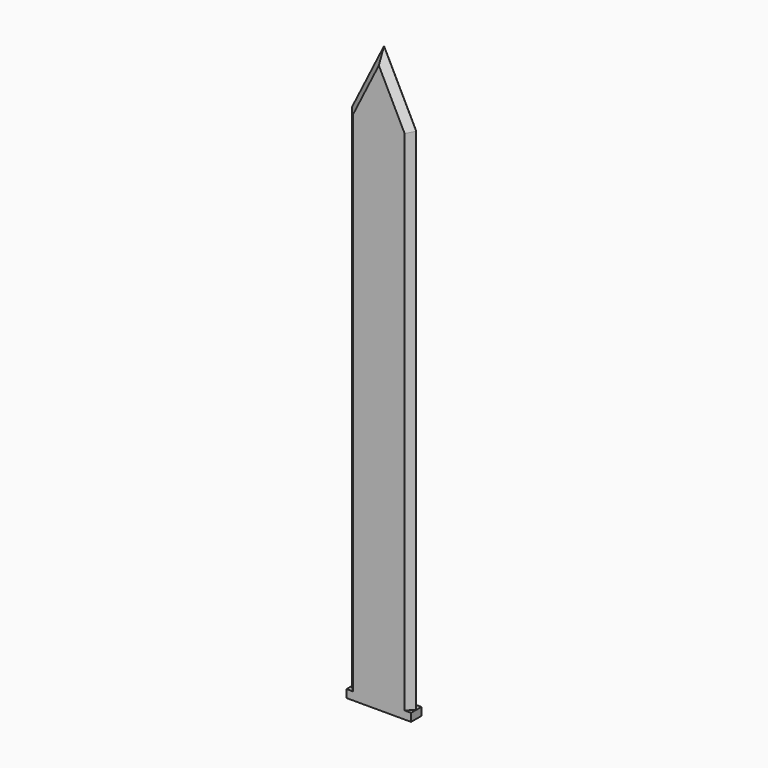
from build123d import *

# Parameters (mm, degrees)
F0_W     = 76.2
F0_H     = 304.8
F1_DEPTH = 7.62
F2_SIZE  = 7.61999
F3_W     = 76.2
F3_H     = 9.4219583702
F4_DEPTH = 15.24


# Not quite as in the source:
# - a fillet or chamfer is up to 0.001 mm smaller than in the source, because OpenCascade refuses the exact size


with BuildPart() as f1:
    # F0 (on Front) → F1 (new body, symmetric)
    with BuildSketch(Plane.XZ):
        with Locations((0, -152.4)):
            Rectangle(F0_W, F0_H)
        with Locations((0, 152.4)):
            Rectangle(F0_W, F0_H)
        Polygon((-38.1, 304.8), (38.1, 304.8), (0, 381), align=None)
    extrude(amount=F1_DEPTH, both=True)

    # F2 (size 7.62 in the source; OpenCascade refuses exactly that, so slightly less here)
    f2_edges = [f1.edges().sort_by_distance(p)[0] for p in [
        (0, -7.62, -304.8),
        (38.1, -7.62, 0),
        (19.05, -7.62, 342.9),
        (-19.05, -7.62, 342.9),
        (-38.1, -7.62, 0),
        (0, 7.62, -304.8),
        (38.1, 7.62, 0),
        (19.05, 7.62, 342.9),
        (-19.05, 7.62, 342.9),
        (-38.1, 7.62, 0),
    ]]
    chamfer(f2_edges, length=F2_SIZE)

    # F3 (on face) → F4 (join)
    with BuildSketch(Plane.XZ.offset(7.62)):
        with Locations((0, -301.8909791851)):
            Rectangle(F3_W, F3_H)
    extrude(amount=-F4_DEPTH)


solid = f1.part
